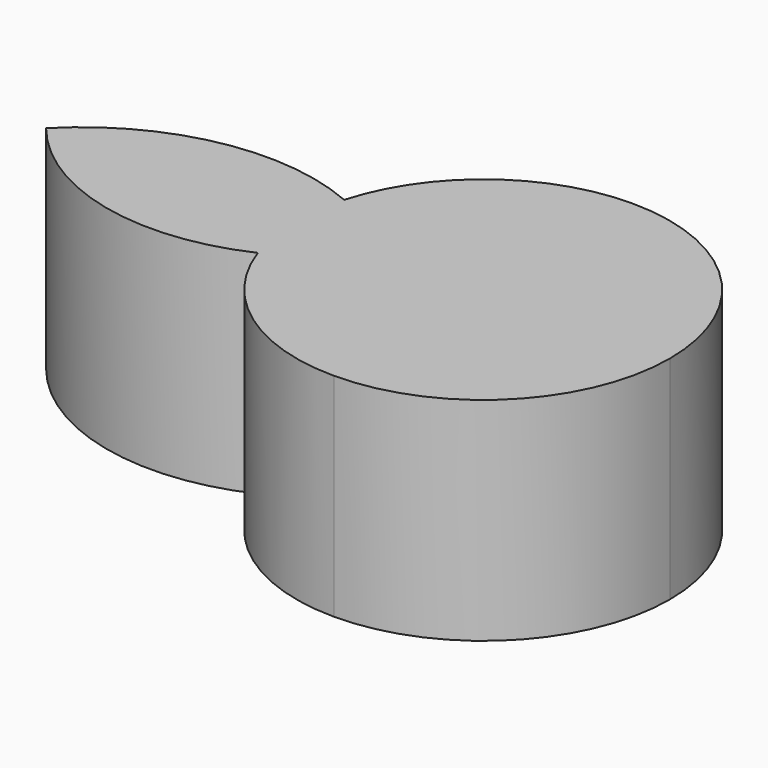
from build123d import *

# Parameters (mm, degrees)
F2_DEPTH = 25.4


# Not quite as in the source:
# - the program builds the solid bodies; features that only make, move or delete a surface that nothing else refers to are left out


with BuildPart() as f2:
    # F0 (on Top) → F2 (new body)
    with BuildSketch(Plane.XY):
        with BuildLine():
            Line((0, -22.3464633732), (0, 0))
            Line((0, 0), (0, 22.3464633732))
            ThreePointArc((0, 22.3464633732), (-13.4819478567, 17.8213778165), (-21.5037952489, 6.0787511204))
            ThreePointArc((-21.5037952489, 6.0787511204), (-22.3364486511, -0.6689446499), (-21.1014820814, -7.354718163))
            ThreePointArc((-21.1014820814, -7.354718163), (-12.9424202767, -18.216975124), (0, -22.3464633732))
        make_face()
        with BuildLine():
            Line((0, 22.3464633732), (0, 0))
            Line((0, 0), (0, -22.3464633732))
            ThreePointArc((0, -22.3464633732), (15.8013357867, -15.8013357867), (22.3464633732, 0))
            ThreePointArc((22.3464633732, 0), (15.8013357867, 15.8013357867), (0, 22.3464633732))
        make_face()
        with BuildLine():
            ThreePointArc((-21.1014820814, -7.354718163), (-22.3364486511, -0.6689446499), (-21.5037952489, 6.0787511204))
            ThreePointArc((-21.5037952489, 6.0787511204), (-37.8621842038, 7.8047564636), (-52.3418858647, 0))
            ThreePointArc((-52.3418858647, 0), (-37.9892096461, -9.0613878034), (-21.1014820814, -7.354718163))
        make_face()
    extrude(amount=F2_DEPTH)


solid = f2.part
